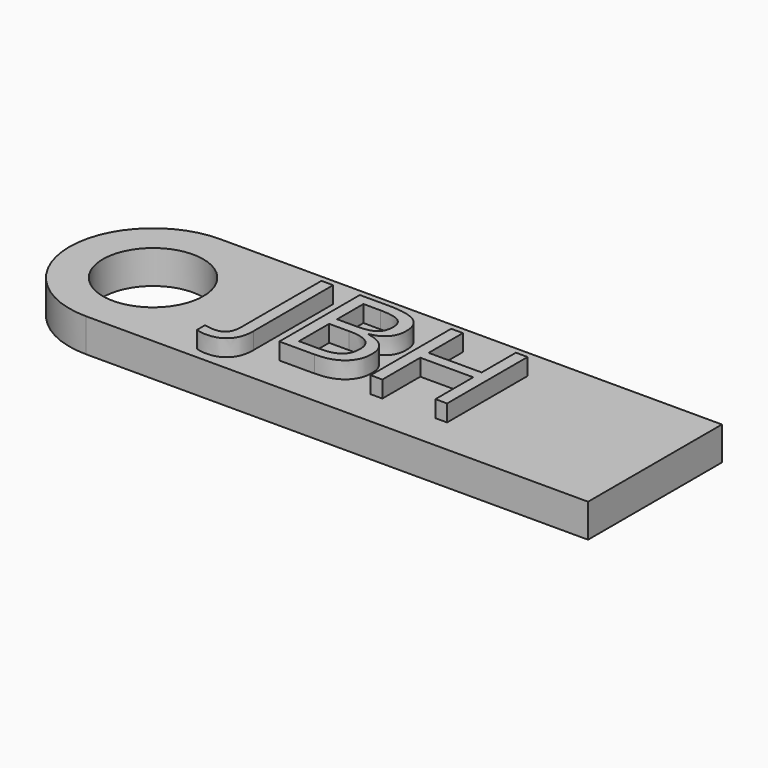
from build123d import *

# Parameters (mm, degrees)
F0_W         = 30
F0_H         = 10
F1_DEPTH     = 2
F2_R         = 3
F3_DEPTH     = 2.5
F4_TEXT_SIZE = 8.4259256255
F5_DEPTH     = 1


# Not quite as in the source:
# - Text() gives the source's letters only with a copy of the font that has no kerning and outlines rounded to 1/6400 em; it was checked with that copy


with BuildPart() as f1:
    # F0 (on Top) → F1 (new body)
    with BuildSketch(Plane.XY):
        with Locations((-30.1367465797, 6.8220342509)):
            Rectangle(F0_W, F0_H)
        with BuildLine():
            Line((-45.1367465797, 1.8220342509), (-45.1367465797, 11.8220342509))
            ThreePointArc((-45.1367465797, 11.8220342509), (-50.1367465797, 6.8220342509), (-45.1367465797, 1.8220342509))
        make_face()
    extrude(amount=F1_DEPTH)

    # F2 (on face) → F3 (cut, symmetric)
    with BuildSketch(Plane.XY.offset(2)):
        with Locations((-45.1367465797, 6.8220342509)):
            Circle(F2_R)
    extrude(amount=F3_DEPTH, both=True, mode=Mode.SUBTRACT)

    # F4 (on face) → F5 (join)
    with BuildSketch(Plane.XY.offset(2)):
        with Locations((-38.3833348751, 3.9666672237)):
            Text('JBH', F4_TEXT_SIZE, font='Open Sans', text_align=(TextAlign.LEFT, TextAlign.BOTTOM))
    extrude(amount=F5_DEPTH)


solid = f1.part
